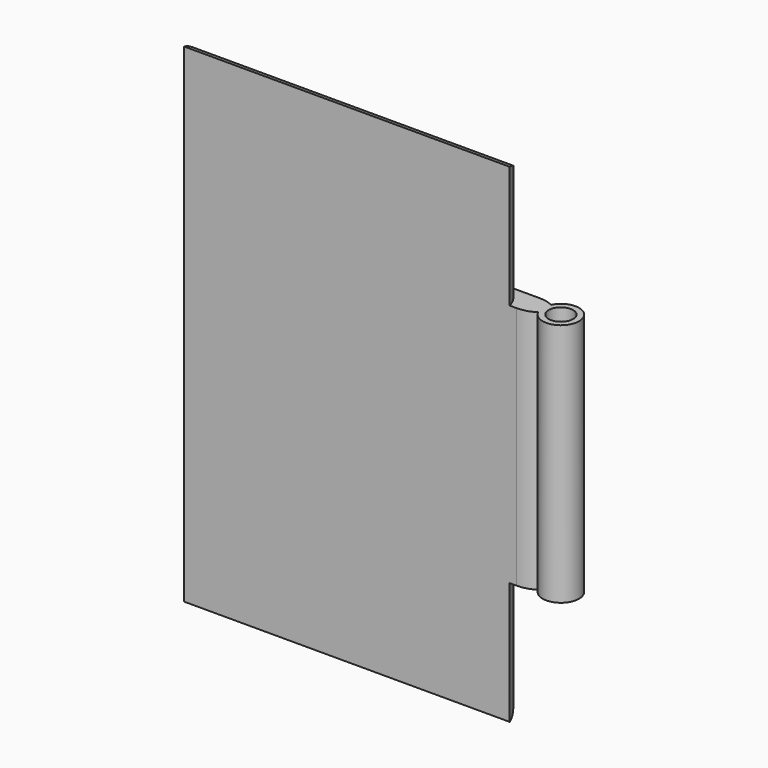
from build123d import *

# Parameters (mm, degrees)
F0_W          = 3.81
F0_H          = 38.1
F1_DEPTH      = 3.81
F2_R          = 2.8295085799
F3_DEPTH      = 19.05
F3_DEPTH_BACK = 19.05
F4_R          = 1.905
F5_DEPTH      = 47.01882
F6_W          = 11.7936587512
F6_H          = 46.736
F7_DEPTH      = 14.81339
F8_W          = 8.9291655459
F8_H          = 39.4763015211
F9_DEPTH      = 25.4
F10_T1_DEPTH  = 11.7936587512
F10_T3_DEPTH  = 11.7936587512
F10_T5_DEPTH  = 11.7936587512
F10_T7_DEPTH  = 11.7936587512
F10_T9_DEPTH  = 39.4763015211
F10_T11_DEPTH = 37.1936587512
F10_T13_DEPTH = 37.1936587512
F10_T15_DEPTH = 39.4763015211
F11_T1_DEPTH  = 75.3934442484
F11_T3_DEPTH  = 31.3467221242
F11_T5_DEPTH  = 31.3467221242
F11_T7_DEPTH  = 49.1322772947
F11_T9_DEPTH  = 51.6998748204


# Not quite as in the source:
# - a fillet or chamfer that OpenCascade refuses, or shapes differently, is made with other operations: its cross-section is extruded or revolved along the edge and cut away or added


with BuildPart() as f1:
    # F0 (on Front) → F1 (new body)
    with BuildSketch(Plane.XZ):
        Polygon((0, 38.1), (-50.8, 38.1), (-50.8, -38.1), (0, -38.1), (0, -19.05), (0, 19.05), align=None)
        with Locations((1.905, 0)):
            Rectangle(F0_W, F0_H)
    extrude(amount=F1_DEPTH)

    # F2 (on Top) → F3 (join, two sides)
    with BuildSketch(Plane.XY) as f3_sk:
        with Locations((6.3444059342, -1.762334723)):
            Circle(F2_R)
    extrude(amount=F3_DEPTH)
    extrude(f3_sk.sketch, amount=-F3_DEPTH_BACK)

    # F4 (on face) → F5 (cut)
    with BuildSketch(Plane.XY.offset(19.05)):
        with Locations((6.3444059342, -1.762334723)):
            Circle(F4_R)
    extrude(amount=-F5_DEPTH, mode=Mode.SUBTRACT)

    # F6 (on face) → F7 (join)
    with BuildSketch(Plane(origin=(0, 0, 0), x_dir=(-1, 0, 0), z_dir=(0, 1, 0))):
        with Locations((44.9031706244, 0)):
            Rectangle(F6_W, F6_H)
    extrude(amount=F7_DEPTH)

    # F8 (on face) → F9 (cut)
    with BuildSketch(Plane(origin=(-50.8, 0, 0), x_dir=(0, -1, 0), z_dir=(-1, 0, 0))):
        with Locations((-6.8143603858, -0.5874447525)):
            Rectangle(F8_W, F8_H)
    extrude(amount=-F9_DEPTH, mode=Mode.SUBTRACT)

    # F10: fillet of radius 5.08 on 8 edges, made by hand

    # F10_s2 → F10_t1 (join)
    with BuildSketch(Plane.YZ.offset(-50.8)):
        with BuildLine():
            ThreePointArc((0, -28.448), (1.4878975516, -24.8558975516), (5.08, -23.368))
            Line((5.08, -23.368), (0, -23.368))
            Line((0, -23.368), (0, -28.448))
        make_face()
    extrude(amount=F10_T1_DEPTH)

    # F10_s4 → F10_t3 (join)
    with BuildSketch(Plane.YZ.offset(-50.8)):
        with BuildLine():
            ThreePointArc((0, 28.448), (1.4878975516, 24.8558975516), (5.08, 23.368))
            Line((5.08, 23.368), (0, 23.368))
            Line((0, 23.368), (0, 28.448))
        make_face()
    extrude(amount=F10_T3_DEPTH)

    # F10_s6 → F10_t5 (join)
    with BuildSketch(Plane.YZ.offset(-50.8)):
        with BuildLine():
            ThreePointArc((11.2789431587, -15.245595513), (9.7910456071, -18.8376979614), (6.1989431587, -20.325595513))
            Line((6.1989431587, -20.325595513), (11.2789431587, -20.325595513))
            Line((11.2789431587, -20.325595513), (11.2789431587, -15.245595513))
        make_face()
    extrude(amount=F10_T5_DEPTH)

    # F10_s8 → F10_t7 (join)
    with BuildSketch(Plane.YZ.offset(-50.8)):
        with BuildLine():
            ThreePointArc((6.1989431587, 19.1507060081), (9.7910456071, 17.6628084565), (11.2789431587, 14.0707060081))
            Line((11.2789431587, 14.0707060081), (11.2789431587, 19.1507060081))
            Line((11.2789431587, 19.1507060081), (6.1989431587, 19.1507060081))
        make_face()
    extrude(amount=F10_T7_DEPTH)

    # F10_s10 → F10_t9 (cut)
    with BuildSketch(Plane.XY.offset(-20.325595513)):
        with BuildLine():
            ThreePointArc((-50.8, -2.7302223872), (-49.3121024484, 0.8618800613), (-45.72, 2.3497776128))
            Line((-45.72, 2.3497776128), (-50.8, 2.3497776128))
            Line((-50.8, 2.3497776128), (-50.8, -2.7302223872))
        make_face()
    extrude(amount=F10_T9_DEPTH, mode=Mode.SUBTRACT)

    # F10_s12 → F10_t11 (cut)
    with BuildSketch(Plane.YZ.offset(-63.5)):
        with BuildLine():
            ThreePointArc((14.81339, 18.288), (13.3254924484, 21.8801024484), (9.73339, 23.368))
            Line((9.73339, 23.368), (14.81339, 23.368))
            Line((14.81339, 23.368), (14.81339, 18.288))
        make_face()
    extrude(amount=F10_T11_DEPTH, mode=Mode.SUBTRACT)

    # F10_s14 → F10_t13 (cut)
    with BuildSketch(Plane.YZ.offset(-63.5)):
        with BuildLine():
            ThreePointArc((14.81339, -18.288), (13.3254924484, -21.8801024484), (9.73339, -23.368))
            Line((9.73339, -23.368), (14.81339, -23.368))
            Line((14.81339, -23.368), (14.81339, -18.288))
        make_face()
    extrude(amount=F10_T13_DEPTH, mode=Mode.SUBTRACT)

    # F10_s16 → F10_t15 (cut)
    with BuildSketch(Plane.XY.offset(-20.325595513)):
        with BuildLine():
            ThreePointArc((-39.0063412488, 0), (-40.8472599359, 1.7237606464), (-43.2902980315, 2.3497776128))
            Line((-43.2902980315, 2.3497776128), (-39.0063412488, 2.3497776128))
            Line((-39.0063412488, 2.3497776128), (-39.0063412488, 0))
        make_face()
    extrude(amount=F10_T15_DEPTH, mode=Mode.SUBTRACT)

    # F11: fillet of radius 5.08 on 6 edges, made by hand

    # F11_s2 → F11_t1 (cut)
    with BuildSketch(Plane.YZ.offset(-63.0967221242)):
        with BuildLine():
            ThreePointArc((0, -33.1813111503), (-1.0639073716, -36.2921631237), (-3.81, -38.1))
            Line((-3.81, -38.1), (0, -38.1))
            Line((0, -38.1), (0, -33.1813111503))
        make_face()
        with BuildLine():
            ThreePointArc((-3.81, 38.1), (-1.0639073716, 36.2921631237), (0, 33.1813111503))
            Line((0, 33.1813111503), (0, 38.1))
            Line((0, 38.1), (-3.81, 38.1))
        make_face()
    extrude(amount=F11_T1_DEPTH, mode=Mode.SUBTRACT)

    # F11_s4 → F11_t3 (cut)
    with BuildSketch(Plane.XY.offset(19.05)):
        with BuildLine():
            ThreePointArc((0, -3.81), (-1.8078368763, -1.0639073716), (-4.9186888497, 0))
            Line((-4.9186888497, 0), (0, 0))
            Line((0, 0), (0, -3.81))
        make_face()
    extrude(amount=F11_T3_DEPTH, mode=Mode.SUBTRACT)

    # F11_s6 → F11_t5 (cut)
    with BuildSketch(Plane.XY.offset(-50.3967221242)):
        with BuildLine():
            ThreePointArc((-4.9186888497, 0), (-1.8078368763, -1.0639073716), (0, -3.81))
            Line((0, -3.81), (0, 0))
            Line((0, 0), (-4.9186888497, 0))
        make_face()
    extrude(amount=F11_T5_DEPTH, mode=Mode.SUBTRACT)

    # F11_s8 → F11_t7 (cut)
    with BuildSketch(Plane.XY.offset(-24.5661386473)):
        with BuildLine():
            ThreePointArc((1.6035445411, 0), (2.7352095066, -0.1276536464), (3.81, -0.5041990529))
            Line((3.81, -0.5041990529), (3.81, 0))
            Line((3.81, 0), (1.6035445411, 0))
        make_face()
    extrude(amount=F11_T7_DEPTH, mode=Mode.SUBTRACT)

    # F11_s10 → F11_t9 (cut)
    with BuildSketch(Plane.XY.offset(-25.8499374102)):
        with BuildLine():
            ThreePointArc((1.0900250359, -3.81), (2.5061483361, -3.6086263229), (3.81, -3.0204703932))
            Line((3.81, -3.0204703932), (3.81, -3.81))
            Line((3.81, -3.81), (1.0900250359, -3.81))
        make_face()
    extrude(amount=F11_T9_DEPTH, mode=Mode.SUBTRACT)


solid = f1.part
